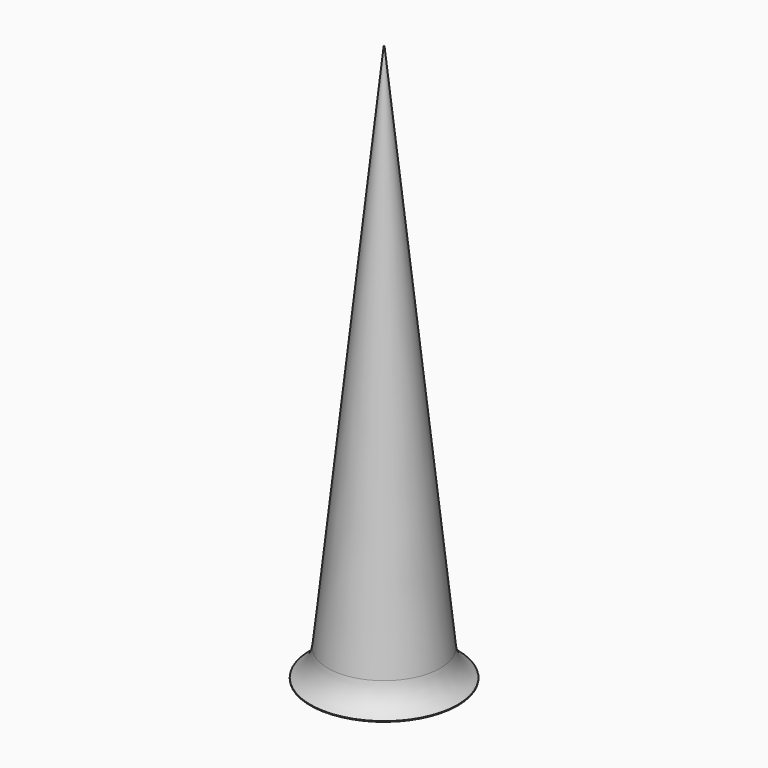
from build123d import *

# Parameters (mm, degrees)
F0_R     = 85
F2_R     = 0.5
F4_R     = 105.9677495378
F5_DEPTH = 1


# Not quite as in the source:
# - a fillet or chamfer that OpenCascade refuses, or shapes differently, is made with other operations: its cross-section is extruded or revolved along the edge and cut away or added


with BuildPart() as f3:
    # F0 (on Top) → F3 section 0
    with BuildSketch(Plane.XY):
        Circle(F0_R)
    # F2 (on offset) → F3 section 1
    with BuildSketch(Plane.XY.offset(800)):
        Circle(F2_R)
    loft()

    # F4 (on Top) → F5 (join)
    with BuildSketch(Plane.XY):
        Circle(F4_R)
    extrude(amount=F5_DEPTH)

    # F6: fillet of radius 50 on 1 edges, made by hand


with BuildPart() as f6_tool2:
    # F6_s3 → F6_t4 (revolve)
    with BuildSketch(Plane.XZ):
        with BuildLine():
            ThreePointArc((105.9675526746, 0.9996517976), (88.7718520485, 17.0936422209), (80.851270192, 39.2741072932))
            Line((80.851270192, 39.2741072932), (75.8787755878, 38.7488875506))
            ThreePointArc((75.8787755878, 38.7488875506), (77.9005268853, 19.6118549121), (79.9218803957, 0.4747802574))
            Line((79.9218803957, 0.4747802574), (84.894375, -4.0001558343))
            ThreePointArc((84.894375, -4.0001558343), (95.4309638373, -4.0001558343), (103.5066863186, -3.3530134945))
            Line((103.5066863186, -3.3530134945), (105.9675526746, 0.9996517976))
        make_face()
    revolve(axis=Axis((0, 0, 1), (0, 0, 1)))

    split(bisect_by=Plane.XY, keep=Keep.TOP)


with BuildPart() as f3_1:
    add(f3.part)

    # F6_t1: union F6_tool2
    add(f6_tool2.part)


solid = f3_1.part
